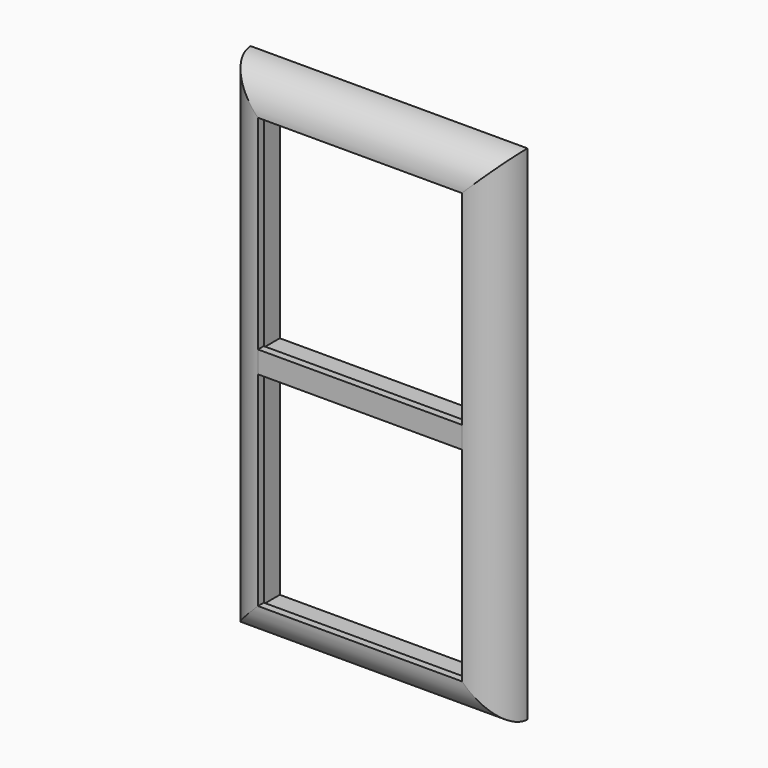
from build123d import *

# Parameters (mm, degrees)
F0_W     = 38
F0_H     = 69
F0_W_2   = 28
F0_H_2   = 28
F0_H_3   = 1
F0_W_3   = 1
F1_DEPTH = 5
F2_DEPTH = 25
F3_DEPTH = 4
F4_R     = 4.99999


# Not quite as in the source:
# - a fillet or chamfer is up to 0.001 mm smaller than in the source, because OpenCascade refuses the exact size


with BuildPart() as f1:
    # F0 (on Front) → F1 (new body)
    with BuildSketch(Plane.XZ):
        Rectangle(F0_W, F0_H)
        Polygon((-15, 0.5), (-15, 1.5), (-15, 30.5), (15, 30.5), (15, 1.5), (15, 0.5), (15, -0.5), (15, -1.5), (15, -30.5), (-15, -30.5), (-15, -1.5), (-15, -0.5), align=None, mode=Mode.SUBTRACT)
        with Locations((0, 15.5)):
            Rectangle(F0_W_2, F0_H_2)
        with Locations((0, -15.5)):
            Rectangle(F0_W_2, F0_H_2)
        Polygon((-14, -29.5), (-14, -1.5), (-15, -1.5), (-15, -30.5), (15, -30.5), (15, -1.5), (14, -1.5), (14, -29.5), align=None)
        Polygon((-14, 1.5), (-14, 29.5), (14, 29.5), (14, 1.5), (15, 1.5), (15, 30.5), (-15, 30.5), (-15, 1.5), align=None)
        with Locations((0, 1)):
            Rectangle(F0_W_2, F0_H_3)
        with Locations((0, -1)):
            Rectangle(F0_W_2, F0_H_3)
        Rectangle(F0_W_2, F0_H_3)
        with Locations((-14.5, 1)):
            Rectangle(F0_W_3, F0_H_3)
        with Locations((-14.5, 0)):
            Rectangle(F0_W_3, F0_H_3)
        with Locations((-14.5, -1)):
            Rectangle(F0_W_3, F0_H_3)
        with Locations((14.5, 1)):
            Rectangle(F0_W_3, F0_H_3)
        with Locations((14.5, 0)):
            Rectangle(F0_W_3, F0_H_3)
        with Locations((14.5, -1)):
            Rectangle(F0_W_3, F0_H_3)
    extrude(amount=F1_DEPTH)

    # F0 (on Front) → F2 (cut)
    with BuildSketch(Plane.XZ):
        with Locations((0, 15.5)):
            Rectangle(F0_W_2, F0_H_2)
        with Locations((0, -15.5)):
            Rectangle(F0_W_2, F0_H_2)
    extrude(amount=F2_DEPTH, mode=Mode.SUBTRACT)

    # F0 (on Front) → F3 (cut)
    with BuildSketch(Plane.XZ):
        Polygon((-14, 1.5), (-14, 29.5), (14, 29.5), (14, 1.5), (15, 1.5), (15, 30.5), (-15, 30.5), (-15, 1.5), align=None)
        with Locations((14.5, 1)):
            Rectangle(F0_W_3, F0_H_3)
        with Locations((0, 1)):
            Rectangle(F0_W_2, F0_H_3)
        with Locations((-14.5, 1)):
            Rectangle(F0_W_3, F0_H_3)
        Polygon((-14, -29.5), (-14, -1.5), (-15, -1.5), (-15, -30.5), (15, -30.5), (15, -1.5), (14, -1.5), (14, -29.5), align=None)
        with Locations((14.5, -1)):
            Rectangle(F0_W_3, F0_H_3)
        with Locations((0, -1)):
            Rectangle(F0_W_2, F0_H_3)
        with Locations((-14.5, -1)):
            Rectangle(F0_W_3, F0_H_3)
    extrude(amount=F3_DEPTH, mode=Mode.SUBTRACT)

    # F4 (radius 5 in the source; OpenCascade refuses exactly that, so slightly less here)
    f4_edges = [f1.edges().sort_by_distance(p)[0] for p in [
        (-19, -5, 0),
        (0, -5, 34.5),
        (19, -5, 0),
        (0, -5, -34.5),
    ]]
    fillet(f4_edges, radius=F4_R)


solid = f1.part
